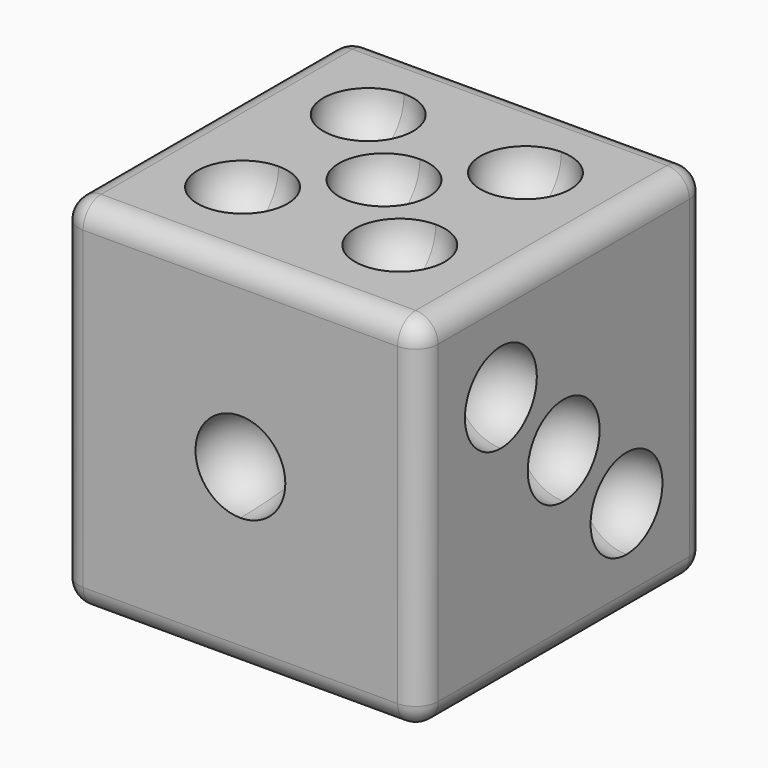
from build123d import *

# Parameters (mm, degrees)
F1_W     = 16
F1_H     = 15.9821804036
F2_DEPTH = 16
F3_R     = 1


# Not quite as in the source:
# - a feature of the source that left no trace in its solid (it failed there, or was rolled back) is left out


with BuildPart() as f2:
    # F1 (on Top) → F2 (new body)
    with BuildSketch(Plane.XY):
        with Locations((8, -7.9910902018)):
            Rectangle(F1_W, F1_H)
    extrude(amount=F2_DEPTH)

    # F3
    f3_edges = [f2.edges().sort_by_distance(p)[0] for p in [
        (0, -7.99109, 16),
        (8, -15.98218, 16),
        (16, -7.99109, 16),
        (8, 0, 16),
        (0, -15.98218, 8),
        (0, 0, 8),
        (16, -15.98218, 8),
        (16, 0, 8),
        (8, 0, 0),
        (0, -7.99109, 0),
        (8, -15.98218, 0),
        (16, -7.99109, 0),
    ]]
    fillet(f3_edges, radius=F3_R)

    # F4 (on face) → F5 (revolve, cut)
    with BuildSketch(Plane.XZ.offset(15.9821804036)):
        with BuildLine():
            ThreePointArc((9.4142135624, 6.5857864376), (9.847759065, 7.2346331353), (10, 8))
            ThreePointArc((10, 8), (8.7653668647, 9.847759065), (6.5857864376, 9.4142135624))
            Line((6.5857864376, 9.4142135624), (9.4142135624, 6.5857864376))
        make_face()
    revolve(axis=Axis((8, -15.9821804036, 8), (0.7071067812, 0, -0.7071067812)), mode=Mode.SUBTRACT)

    # F6 (on face) → F7 (revolve, cut)
    with BuildSketch(Plane(origin=(0, 0, 0), x_dir=(-1, 0, 0), z_dir=(0, 1, 0))):
        with BuildLine():
            ThreePointArc((-6, 8), (-7.2346331353, 9.847759065), (-9.4142135624, 9.4142135624))
            Line((-9.4142135624, 9.4142135624), (-6.5857864376, 6.5857864376))
            ThreePointArc((-6.5857864376, 6.5857864376), (-6.152240935, 7.2346331353), (-6, 8))
        make_face()
    revolve(axis=Axis((8, 0, 8), (-0.7071067812, 0, -0.7071067812)), mode=Mode.SUBTRACT)

    # F8 (on face) → F9 (revolve, cut)
    with BuildSketch(Plane(origin=(0, 0, 0), x_dir=(0, -1, 0), z_dir=(-1, 0, 0))):
        with BuildLine():
            Line((4.4955451009, 11.5), (4.4955451009, 13.5))
            ThreePointArc((4.4955451009, 13.5), (3.0813315385, 12.9142135624), (2.4955451009, 11.5))
            Line((2.4955451009, 11.5), (4.4955451009, 11.5))
        make_face()
        with BuildLine():
            Line((4.4955451009, 11.5), (6.4955451009, 11.5))
            ThreePointArc((6.4955451009, 11.5), (5.9097586633, 12.9142135624), (4.4955451009, 13.5))
            Line((4.4955451009, 13.5), (4.4955451009, 11.5))
        make_face()
    revolve(axis=Axis((0, -7.9910902018, 11.5), (0, -1, 0)), mode=Mode.SUBTRACT)

    # F8 (on face) → F10 (revolve, cut)
    with BuildSketch(Plane(origin=(0, 0, 0), x_dir=(0, -1, 0), z_dir=(-1, 0, 0))):
        with BuildLine():
            Line((11.4866353027, 4.5), (9.4866353027, 4.5))
            ThreePointArc((9.4866353027, 4.5), (10.0724217403, 3.0857864376), (11.4866353027, 2.5))
            Line((11.4866353027, 2.5), (11.4866353027, 4.5))
        make_face()
        with BuildLine():
            Line((11.4866353027, 4.5), (11.4866353027, 2.5))
            ThreePointArc((11.4866353027, 2.5), (12.9008488651, 3.0857864376), (13.4866353027, 4.5))
            Line((13.4866353027, 4.5), (11.4866353027, 4.5))
        make_face()
    revolve(axis=Axis((0, -7.9910902018, 4.5), (0, -1, 0)), mode=Mode.SUBTRACT)

    # F11 (on face) → F12 (revolve, cut)
    with BuildSketch(Plane.YZ.offset(16)):
        with BuildLine():
            Line((-11.4866353027, 11.5), (-11.4866353027, 13.5))
            ThreePointArc((-11.4866353027, 13.5), (-12.9008488651, 12.9142135624), (-13.4866353027, 11.5))
            Line((-13.4866353027, 11.5), (-11.4866353027, 11.5))
        make_face()
        with BuildLine():
            Line((-11.4866353027, 11.5), (-9.4866353027, 11.5))
            ThreePointArc((-9.4866353027, 11.5), (-10.0724217403, 12.9142135624), (-11.4866353027, 13.5))
            Line((-11.4866353027, 13.5), (-11.4866353027, 11.5))
        make_face()
    revolve(axis=Axis((16, -7.9910902018, 11.5), (0, -1, 0)), mode=Mode.SUBTRACT)

    # F11 (on face) → F13 (revolve, cut)
    with BuildSketch(Plane.YZ.offset(16)):
        with BuildLine():
            Line((-7.9910902018, 8), (-7.9910902018, 10))
            ThreePointArc((-7.9910902018, 10), (-9.4053037642, 9.4142135624), (-9.9910902018, 8))
            Line((-9.9910902018, 8), (-7.9910902018, 8))
        make_face()
        with BuildLine():
            ThreePointArc((-5.9910902018, 8), (-6.5768766394, 9.4142135624), (-7.9910902018, 10))
            Line((-7.9910902018, 10), (-7.9910902018, 8))
            Line((-7.9910902018, 8), (-5.9910902018, 8))
        make_face()
    revolve(axis=Axis((16, -4.4955451009, 8), (0, 1, 0)), mode=Mode.SUBTRACT)

    # F11 (on face) → F14 (revolve, cut)
    with BuildSketch(Plane.YZ.offset(16)):
        with BuildLine():
            Line((-4.4955451009, 4.5), (-4.4955451009, 6.5))
            ThreePointArc((-4.4955451009, 6.5), (-5.9097586633, 5.9142135624), (-6.4955451009, 4.5))
            Line((-6.4955451009, 4.5), (-4.4955451009, 4.5))
        make_face()
        with BuildLine():
            ThreePointArc((-2.4955451009, 4.5), (-3.0813315385, 5.9142135624), (-4.4955451009, 6.5))
            Line((-4.4955451009, 6.5), (-4.4955451009, 4.5))
            Line((-4.4955451009, 4.5), (-2.4955451009, 4.5))
        make_face()
    revolve(axis=Axis((16, -7.9910902018, 4.5), (0, 1, 0)), mode=Mode.SUBTRACT)

    # F15 (on face) → F16 (revolve, cut)
    with BuildSketch(Plane.XY.offset(16)):
        with BuildLine():
            ThreePointArc((4.5, -2.4955451009), (3.0857864376, -3.0813315385), (2.5, -4.4955451009))
            Line((2.5, -4.4955451009), (4.5, -4.4955451009))
            Line((4.5, -4.4955451009), (4.5, -2.4955451009))
        make_face()
        with BuildLine():
            Line((4.5, -2.4955451009), (4.5, -4.4955451009))
            Line((4.5, -4.4955451009), (6.5, -4.4955451009))
            ThreePointArc((6.5, -4.4955451009), (5.9142135624, -3.0813315385), (4.5, -2.4955451009))
        make_face()
        with BuildLine():
            ThreePointArc((11.5, -2.4955451009), (10.0857864376, -3.0813315385), (9.5, -4.4955451009))
            Line((9.5, -4.4955451009), (11.5, -4.4955451009))
            Line((11.5, -4.4955451009), (11.5, -2.4955451009))
        make_face()
        with BuildLine():
            ThreePointArc((13.5, -4.4955451009), (12.9142135624, -3.0813315385), (11.5, -2.4955451009))
            Line((11.5, -2.4955451009), (11.5, -4.4955451009))
            Line((11.5, -4.4955451009), (13.5, -4.4955451009))
        make_face()
    revolve(axis=Axis((8, -4.4955451009, 16), (1, 0, 0)), mode=Mode.SUBTRACT)

    # F15 (on face) → F17 (revolve, cut)
    with BuildSketch(Plane.XY.offset(16)):
        with BuildLine():
            ThreePointArc((4.5, -9.4866353027), (3.0857864376, -10.0724217403), (2.5, -11.4866353027))
            Line((2.5, -11.4866353027), (4.5, -11.4866353027))
            Line((4.5, -11.4866353027), (4.5, -9.4866353027))
        make_face()
        with BuildLine():
            Line((4.5, -9.4866353027), (4.5, -11.4866353027))
            Line((4.5, -11.4866353027), (6.5, -11.4866353027))
            ThreePointArc((6.5, -11.4866353027), (5.9142135624, -10.0724217403), (4.5, -9.4866353027))
        make_face()
        with BuildLine():
            ThreePointArc((11.5, -9.4866353027), (10.0857864376, -10.0724217403), (9.5, -11.4866353027))
            Line((9.5, -11.4866353027), (11.5, -11.4866353027))
            Line((11.5, -11.4866353027), (11.5, -9.4866353027))
        make_face()
        with BuildLine():
            Line((11.5, -9.4866353027), (11.5, -11.4866353027))
            Line((11.5, -11.4866353027), (13.5, -11.4866353027))
            ThreePointArc((13.5, -11.4866353027), (12.9142135624, -10.0724217403), (11.5, -9.4866353027))
        make_face()
    revolve(axis=Axis((8, -11.4866353027, 16), (1, 0, 0)), mode=Mode.SUBTRACT)

    # F15 (on face) → F18 (revolve, cut)
    with BuildSketch(Plane.XY.offset(16)):
        with BuildLine():
            ThreePointArc((8, -5.9910902018), (6.5857864376, -6.5768766394), (6, -7.9910902018))
            Line((6, -7.9910902018), (8, -7.9910902018))
            Line((8, -7.9910902018), (8, -5.9910902018))
        make_face()
        with BuildLine():
            Line((8, -5.9910902018), (8, -7.9910902018))
            Line((8, -7.9910902018), (10, -7.9910902018))
            ThreePointArc((10, -7.9910902018), (9.4142135624, -6.5768766394), (8, -5.9910902018))
        make_face()
    revolve(axis=Axis((8, -7.9910902018, 16), (1, 0, 0)), mode=Mode.SUBTRACT)


solid = f2.part
